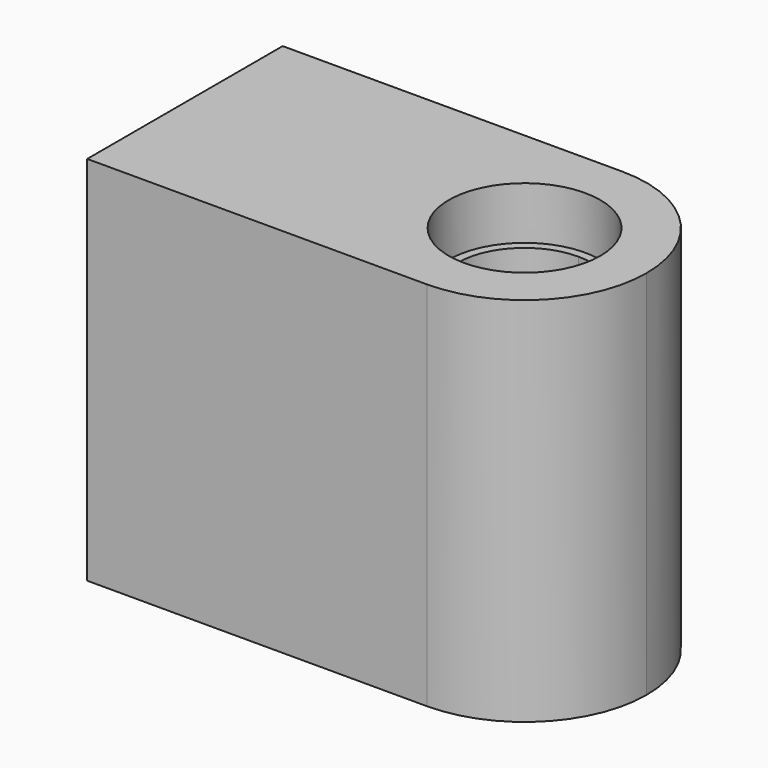
from build123d import *

# Parameters (mm, degrees)
F1_DEPTH = 30.4
F2_W     = 6.8
F2_H     = 6.8
F3_DEPTH = 50
F4_R     = 6.2
F4_R_2   = 5.5
F5_DEPTH = 4.3
F6_DEPTH = 4.3
F7_DEPTH = 2


# Not quite as in the source:
# - a feature names something its author has since deleted; it is built from what else it names


with BuildPart() as f1:
    # F0 (on Top) → F1 (new body)
    with BuildSketch(Plane.XY):
        with BuildLine():
            ThreePointArc((0, -10), (-10, 0), (0, 10))
            Line((0, 10), (-27.8, 10))
            Line((-27.8, 10), (-27.8, -10))
            Line((-27.8, -10), (0, -10))
        make_face()
        with BuildLine():
            ThreePointArc((0, -10), (7.0710678119, -7.0710678119), (10, 0))
            ThreePointArc((10, 0), (7.0710678119, 7.0710678119), (0, 10))
            Line((0, 10), (0, 6.2))
            ThreePointArc((0, 6.2), (4.3840620434, 4.3840620434), (6.2, 0))
            ThreePointArc((6.2, 0), (4.3840620434, -4.3840620434), (0, -6.2))
            Line((0, -6.2), (0, -10))
        make_face()
        with BuildLine():
            Line((0, 6.2), (0, 10))
            ThreePointArc((0, 10), (-10, 0), (0, -10))
            Line((0, -10), (0, -6.2))
            ThreePointArc((0, -6.2), (-6.2, 0), (0, 6.2))
        make_face()
        with BuildLine():
            Line((0, 5.5), (0, 6.2))
            ThreePointArc((0, 6.2), (-6.2, 0), (0, -6.2))
            Line((0, -6.2), (0, -5.5))
            ThreePointArc((0, -5.5), (-5.5, 0), (0, 5.5))
        make_face()
        with BuildLine():
            ThreePointArc((6.2, 0), (4.3840620434, 4.3840620434), (0, 6.2))
            Line((0, 6.2), (0, 5.5))
            ThreePointArc((0, 5.5), (3.8890872965, 3.8890872965), (5.5, 0))
            ThreePointArc((5.5, 0), (3.8890872965, -3.8890872965), (0, -5.5))
            Line((0, -5.5), (0, -6.2))
            ThreePointArc((0, -6.2), (4.3840620434, -4.3840620434), (6.2, 0))
        make_face()
    extrude(amount=F1_DEPTH)

    # F2 (on face) → F3 (cut)
    with BuildSketch(Plane.XZ.offset(10)):
        with Locations((-22.4, 25)):
            Rectangle(F2_W, F2_H)
        with Locations((-22.4, 5.4)):
            Rectangle(F2_W, F2_H)
    extrude(amount=-F3_DEPTH, mode=Mode.SUBTRACT)

    # F4 (on face) → F5 (cut)
    with BuildSketch(Plane.XY.offset(30.4)):
        Circle(F4_R)
        Circle(F4_R_2, mode=Mode.SUBTRACT)
    extrude(amount=-F5_DEPTH, mode=Mode.SUBTRACT)

    # F0 (on Top) → F6 (cut)
    with BuildSketch(Plane.XY):
        with BuildLine():
            ThreePointArc((6.2, 0), (4.3840620434, 4.3840620434), (0, 6.2))
            Line((0, 6.2), (0, 5.5))
            ThreePointArc((0, 5.5), (3.8890872965, 3.8890872965), (5.5, 0))
            ThreePointArc((5.5, 0), (3.8890872965, -3.8890872965), (0, -5.5))
            Line((0, -5.5), (0, -6.2))
            ThreePointArc((0, -6.2), (4.3840620434, -4.3840620434), (6.2, 0))
        make_face()
        with BuildLine():
            Line((0, 5.5), (0, 6.2))
            ThreePointArc((0, 6.2), (-6.2, 0), (0, -6.2))
            Line((0, -6.2), (0, -5.5))
            ThreePointArc((0, -5.5), (-5.5, 0), (0, 5.5))
        make_face()
    extrude(amount=F6_DEPTH, mode=Mode.SUBTRACT)

    # F2 (on face) → F7 (join)
    with BuildSketch(Plane.XZ.offset(10)):
        with Locations((-22.4, 25)):
            Rectangle(F2_W, F2_H)
        with Locations((-22.4, 5.4)):
            Rectangle(F2_W, F2_H)
    extrude(amount=-F7_DEPTH)


solid = f1.part
